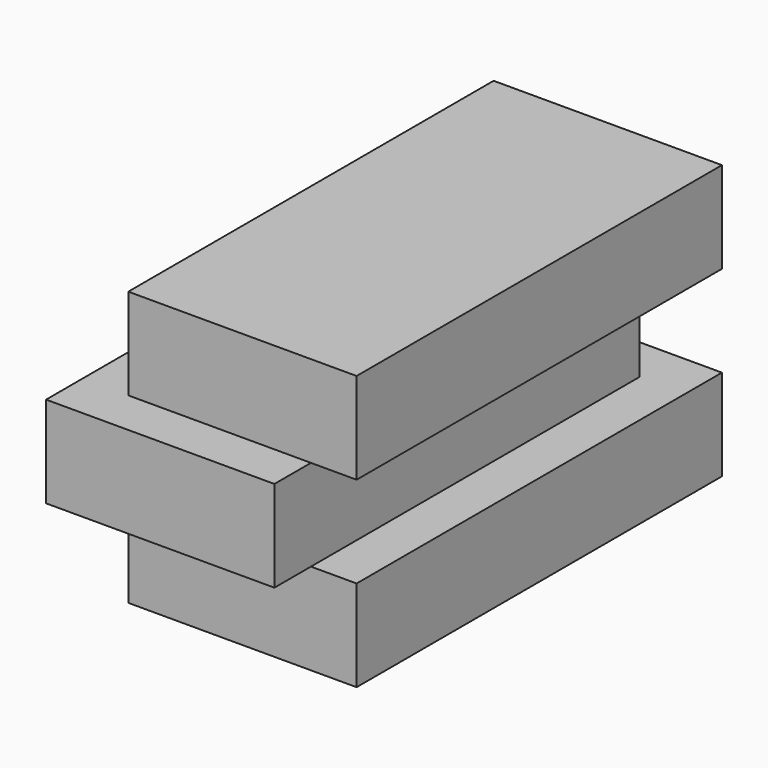
from build123d import *

# Parameters (mm, degrees)
F2_W     = 7.9375
F2_H     = 15.875
F3_DEPTH = 3.175
F4_W     = 7.9375
F4_H     = 15.875
F5_DEPTH = 3.175
F6_W     = 7.9375
F6_H     = 15.875
F7_DEPTH = 3.175


# Not quite as in the source:
# - a variable given as a bare number and used for a length is read in inches; the dataset says mm whatever the document's units were


with BuildPart() as f3:
    # F2 (on Top) → F3 (new body)
    with BuildSketch(Plane.XY):
        with Locations((3.96875, 7.9375)):
            Rectangle(F2_W, F2_H)
    extrude(amount=F3_DEPTH)

    # F4 (on face) → F5 (join)
    with BuildSketch(Plane.XY.offset(3.175)):
        with Locations((2.38125, 6.35)):
            Rectangle(F4_W, F4_H)
    extrude(amount=F5_DEPTH)

    # F6 (on face) → F7 (join)
    with BuildSketch(Plane.XY.offset(6.35)):
        with Locations((3.96875, 7.9375)):
            Rectangle(F6_W, F6_H)
    extrude(amount=F7_DEPTH)


solid = f3.part
